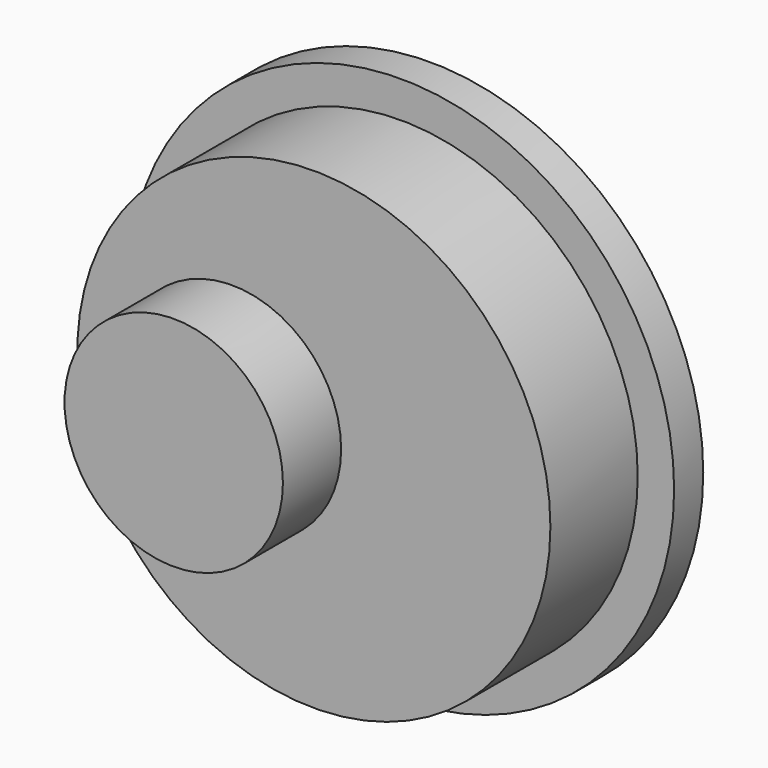
from build123d import *

# Parameters (mm, degrees)
F0_R     = 11.90625
F1_DEPTH = 1.5875
F2_R     = 10.31875
F3_DEPTH = 4.7625
F4_R     = 4.7625
F5_DEPTH = 3.175


# Not quite as in the source:
# - a length typed as a fraction of an inch, garbled in the dataset ("3 / 203.2 mm" for 3/8 in), is restored


with BuildPart() as f1:
    # F0 (on Front) → F1 (new body)
    with BuildSketch(Plane.XZ):
        Circle(F0_R)
    extrude(amount=F1_DEPTH)

    # F2 (on face) → F3 (join)
    with BuildSketch(Plane.XZ.offset(1.5875)):
        Circle(F2_R)
    extrude(amount=F3_DEPTH)

    # F4 (on face) → F5 (join)
    with BuildSketch(Plane.XZ.offset(6.35)):
        with Locations((-3.571875, 0)):
            Circle(F4_R)
    extrude(amount=F5_DEPTH)


solid = f1.part
